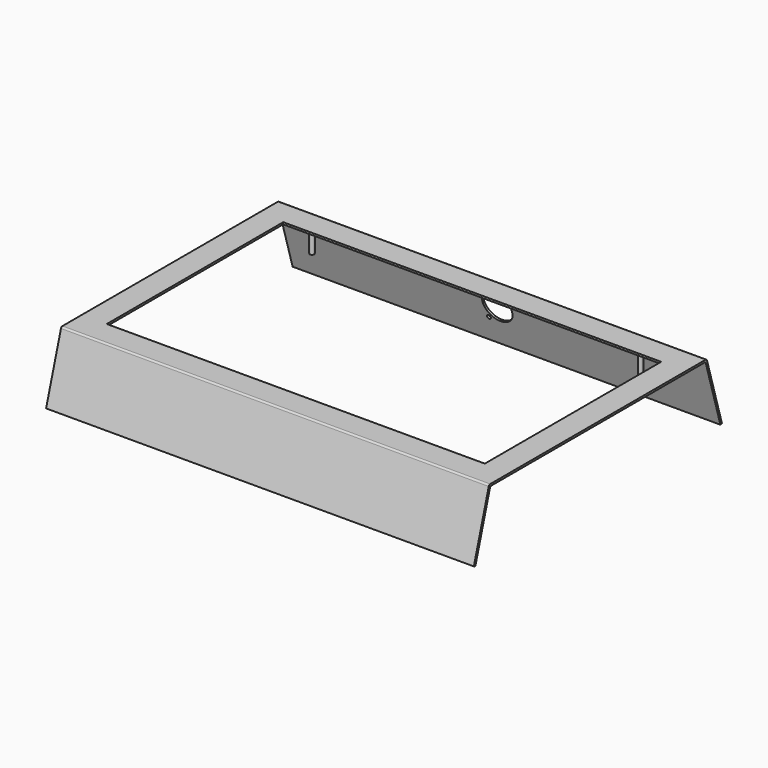
from build123d import *

# Parameters (mm, degrees)
F1_DEPTH = 172.466
F2_W     = 304.8
F2_H     = 177.8
F3_DEPTH = 12.7
F5_R     = 1.75
F6_DEPTH = 15.875
F7_D     = 3.3
F8_D     = 3.3
F9_D     = 24


# Not quite as in the source:
# - a length typed as a fraction of an inch, garbled in the dataset ("3 / 203.2 mm" for 3/8 in), is restored


with BuildPart() as f1:
    # F0 (on Right) → F1 (new body, symmetric)
    with BuildSketch(Plane.YZ):
        with BuildLine():
            Line((-120.2458515259, 50.6342471194), (-135.2673108323, 0))
            Line((-135.2673108323, 0), (-133.7458515259, -0.4513652391))
            Line((-133.7458515259, -0.4513652391), (-119.0612964359, 49.0472471194))
            ThreePointArc((-119.0612964359, 49.0472471194), (-118.4891137925, 49.8676691335), (-117.5398371295, 50.1828818803))
            Line((-117.5398371295, 50.1828818803), (97.0481340778, 50.1828818803))
            ThreePointArc((97.0481340778, 50.1828818803), (97.9974107407, 49.8676691335), (98.5695933841, 49.0472471194))
            Line((98.5695933841, 49.0472471194), (113.2541484741, -0.4513652391))
            Line((113.2541484741, -0.4513652391), (114.7756077805, 0))
            Line((114.7756077805, 0), (99.7541484741, 50.6342471194))
            ThreePointArc((99.7541484741, 50.6342471194), (99.1819658307, 51.4546691335), (98.2326891677, 51.7698818803))
            Line((98.2326891677, 51.7698818803), (-118.7243922195, 51.7698818803))
            ThreePointArc((-118.7243922195, 51.7698818803), (-119.6736688824, 51.4546691335), (-120.2458515259, 50.6342471194))
        make_face()
    extrude(amount=F1_DEPTH, both=True)

    # F2 (on face) → F3 (cut, symmetric)
    with BuildSketch(Plane.XY.offset(51.7698818803)):
        with Locations((0, -10.2458515259)):
            Rectangle(F2_W, F2_H)
    extrude(amount=F3_DEPTH, both=True, mode=Mode.SUBTRACT)

    # F5 (on face) → F6 (join)
    with BuildSketch(Plane(origin=(0, 0, 50.1828818803), x_dir=(1, 0, 0), z_dir=(0, 0, -1))):
        with Locations((132.466, -82.7541484741)):
            Circle(F5_R)
        with Locations((132.466, 103.2458515259)):
            Circle(F5_R)
        with Locations((-132.466, 103.2458515259)):
            Circle(F5_R)
        with Locations((-132.466, -82.7541484741)):
            Circle(F5_R)
    extrude(amount=F6_DEPTH)

    # F7 (through all)
    with Locations(Plane(origin=(0, 105.4912478783, 31.2956660231), x_dir=(-1, 0, 0), z_dir=(0, 0.9587015163, 0.2844141393))):
        with Locations((-9.5, 12)):
            Hole(F7_D / 2)

    # F8 (through all)
    with Locations(Plane(origin=(0, 105.4912478783, 31.2956660231), x_dir=(-1, 0, 0), z_dir=(0, 0.9587015163, 0.2844141393))):
        with Locations((9.5, -12)):
            Hole(F8_D / 2)

    # F9 (through all)
    with Locations(Plane(origin=(0, 105.4912478783, 31.2956660231), x_dir=(-1, 0, 0), z_dir=(0, 0.9587015163, 0.2844141393))):
        with Locations((0, 0)):
            Hole(F9_D / 2)


solid = f1.part
